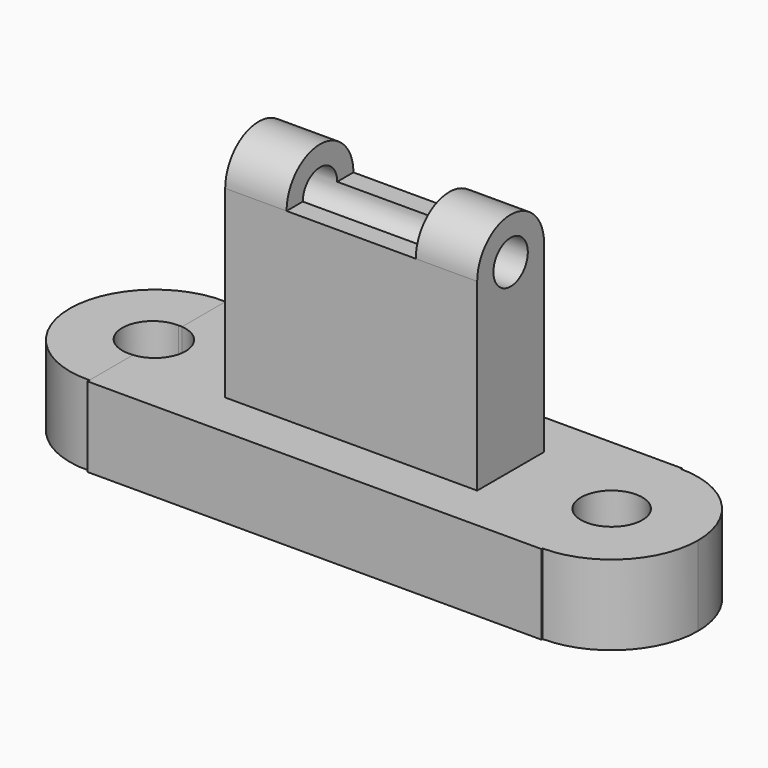
from build123d import *

# Parameters (mm, degrees)
F4_DEPTH  = 16.51
F6_DEPTH  = 16.51
F7_D      = 12.7
F8_D      = 12.7
F9_D      = 12.7
F9_2_D    = 12.7
F10_W     = 52.1319508553
F10_H     = 17.2843895853
F11_DEPTH = 38.1
F13_DEPTH = 12.7
F15_DEPTH = 12.7
F17_D     = 8.89


# Not quite as in the source:
# - the program builds the solid bodies; features that only make, move or delete a surface that nothing else refers to are left out


with BuildPart() as f4:
    # F1 (on face) → F4 (new body)
    with BuildSketch(Plane.XY):
        with BuildLine():
            ThreePointArc((46.9745136797, -17.8288787387), (29.1456349411, 0), (46.9745136797, 17.8288787387))
            Line((46.9745136797, 17.8288787387), (46.9745136797, 18.1207321584))
            Line((46.9745136797, 18.1207321584), (-46.9745136797, 18.1207321584))
            Line((-46.9745136797, 18.1207321584), (-46.9745136797, -18.1207321584))
            Line((-46.9745136797, -18.1207321584), (46.9745136797, -18.1207321584))
            Line((46.9745136797, -18.1207321584), (46.9745136797, -17.8288787387))
        make_face()
    extrude(amount=F4_DEPTH)

    # F1 (on face) → F6 (join)
    with BuildSketch(Plane.XY):
        with BuildLine():
            ThreePointArc((46.9745136797, -17.8288787387), (59.5814347368, -12.6069210571), (64.8033924184, 0))
            ThreePointArc((64.8033924184, 0), (59.5814347368, 12.6069210571), (46.9745136797, 17.8288787387))
            Line((46.9745136797, 17.8288787387), (46.9745136797, -17.8288787387))
        make_face()
        with BuildLine():
            Line((46.9745136797, -17.8288787387), (46.9745136797, 17.8288787387))
            ThreePointArc((46.9745136797, 17.8288787387), (29.1456349411, 0), (46.9745136797, -17.8288787387))
        make_face()
    extrude(amount=F6_DEPTH)

    # F8 (through all)
    with Locations(Plane(origin=(0, 0, 0), x_dir=(1, 0, 0), z_dir=(0, 0, -1))):
        with Locations((46.9745136797, 0)):
            Hole(F8_D / 2)

    # F9 (through all)
    with Locations(Plane(origin=(0, 0, 0), x_dir=(1, 0, 0), z_dir=(0, 0, -1))):
        with Locations((-47.5320741534, 0)):
            Hole(F9_D / 2)

    # F10 (on face) → F11 (join)
    with BuildSketch(Plane.XY.offset(16.51)):
        Rectangle(F10_W, F10_H)
    extrude(amount=F11_DEPTH)

    # F12 (on face) → F13 (join)
    with BuildSketch(Plane(origin=(-26.0659754276, 0, 0), x_dir=(0, -1, 0), z_dir=(-1, 0, 0))):
        with BuildLine():
            Line((-8.6421947926, 54.61), (8.6421947926, 54.61))
            ThreePointArc((8.6421947926, 54.61), (0, 63.2521947926), (-8.6421947926, 54.61))
        make_face()
    extrude(amount=-F13_DEPTH)

    # F14 (on face) → F15 (join)
    with BuildSketch(Plane.YZ.offset(26.0659754276)):
        with BuildLine():
            Line((-8.6421947926, 54.61), (8.6421947926, 54.61))
            ThreePointArc((8.6421947926, 54.61), (0, 63.2521947926), (-8.6421947926, 54.61))
        make_face()
    extrude(amount=-F15_DEPTH)

    # F17 (through all)
    with Locations(Plane.YZ.offset(26.0659754276)):
        with Locations((0, 54.61)):
            Hole(F17_D / 2)


with BuildPart() as f4b:
    # F2 (on face) → F4, piece 2 (new body)
    with BuildSketch(Plane.XY):
        with BuildLine():
            Line((-46.9745136797, -17.5897021865), (-46.9745136797, 17.5897021865))
            ThreePointArc((-46.9745136797, 17.5897021865), (-65.1306109304, 0), (-46.9745136797, -17.5897021865))
        make_face()
    extrude(amount=F4_DEPTH)

    # F7 (through all)
    with Locations(Plane(origin=(0, 0, 0), x_dir=(1, 0, 0), z_dir=(0, 0, -1))):
        with Locations((-47.9283444583, 0)):
            Hole(F7_D / 2)

    # F9#2 (through all)
    with Locations(Plane(origin=(0, 0, 0), x_dir=(1, 0, 0), z_dir=(0, 0, -1))):
        with Locations((-47.5320741534, 0)):
            Hole(F9_2_D / 2)


solid = Compound([f4.part, f4b.part])
